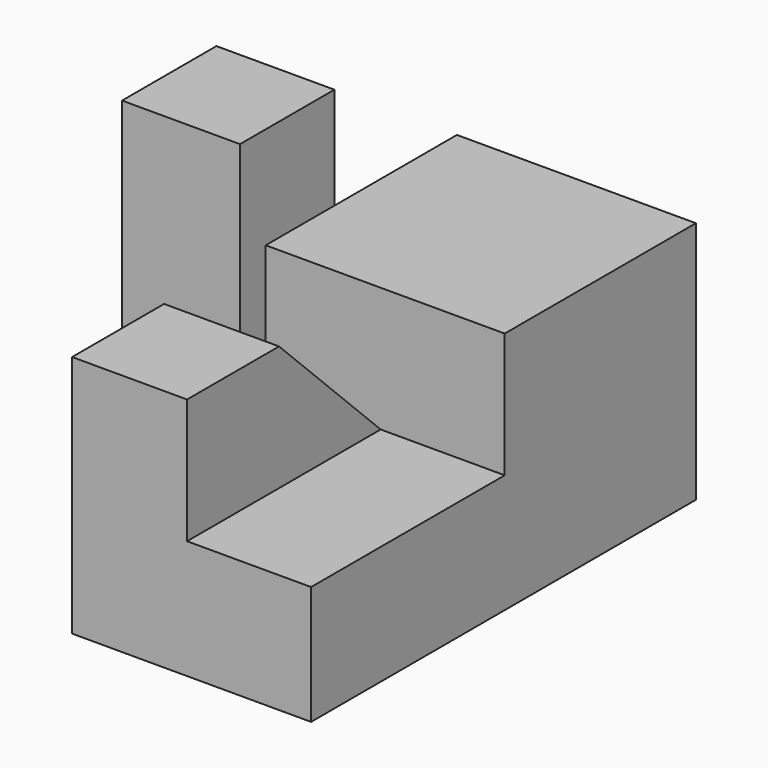
from build123d import *

# Parameters (mm, degrees)
F0_W      = 15.8
F0_H      = 15.8
F1_DEPTH  = 16.1
F3_DEPTH  = 8.1
F5_DEPTH  = 7.8
F6_W      = 15.8
F6_H      = 16
F7_DEPTH  = 7.85
F8_W      = 7.6
F8_H      = 7.6
F9_DEPTH  = 8.25
F11_DEPTH = 7.6
F13_W     = 7.8
F13_H     = 7.8
F14_DEPTH = 25.4


with BuildPart() as f1:
    # F0 (on Top) → F1 (new body)
    with BuildSketch(Plane.XY):
        with Locations((-0.699278047, -1.1891025347)):
            Rectangle(F0_W, F0_H)
    extrude(amount=F1_DEPTH)

    # F2 (on face) → F3 (join)
    with BuildSketch(Plane(origin=(-8.599278047, 0, 0), x_dir=(0, -1, 0), z_dir=(-1, 0, 0))):
        Polygon((1.2891025347, 0), (9.0891025347, 0), (9.0891025347, 8.2), align=None)
    extrude(amount=F3_DEPTH)

    # F4 (on face) → F5 (join)
    with BuildSketch(Plane(origin=(-16.699278047, 0, 0), x_dir=(0, -1, 0), z_dir=(-1, 0, 0))):
        Polygon((1.2891025347, 16.1), (1.2891025347, 0), (9.0891025347, 8.2), (9.0891025347, 16.1), align=None)
        Polygon((1.2891025347, 0), (9.0891025347, 0), (9.0891025347, 8.2), align=None)
    extrude(amount=F5_DEPTH)

    # F6 (on face) → F7 (join)
    with BuildSketch(Plane(origin=(0, 0, 0), x_dir=(1, 0, 0), z_dir=(0, 0, -1))):
        with Locations((-0.699278047, -14.7108974653)):
            Rectangle(F6_W, F6_H)
    extrude(amount=-F7_DEPTH)

    # F8 (on face) → F9 (join, through all)
    with BuildSketch(Plane.XY.offset(7.85)):
        with Locations((-4.799278047, 18.9108974653)):
            Rectangle(F8_W, F8_H)
    extrude(amount=F9_DEPTH)

    # F10 (on face) → F11 (join, through all)
    with BuildSketch(Plane(origin=(-8.599278047, 0, 0), x_dir=(0, -1, 0), z_dir=(-1, 0, 0))):
        Polygon((-6.7108974653, 7.85), (-15.1108974653, 16.1), (-15.1108974653, 7.85), align=None)
    extrude(amount=-F11_DEPTH)

    # F12: F1 across face


with BuildPart() as f1_1:
    add(f1.part)
    add(f1.part.mirror(Plane(origin=(-8.0758652597, -9.0891025347, 7.462251893), x_dir=(1, 0, 0), z_dir=(0, -1, 0))))

    # F13 (on face) → F14 (cut)
    with BuildSketch(Plane.XY.offset(16.1)):
        with Locations((-20.599278047, -5.1891025347)):
            Rectangle(F13_W, F13_H)
        Polygon((-16.699278047, -1.2891025347), (-16.699278047, -9.0891025347), (7.200721953, -9.0891025347), (7.200721953, 22.7108974653), (-24.499278047, 22.7108974653), (-24.499278047, -1.2891025347), align=None)
    extrude(amount=-F14_DEPTH, mode=Mode.SUBTRACT)


solid = f1_1.part
